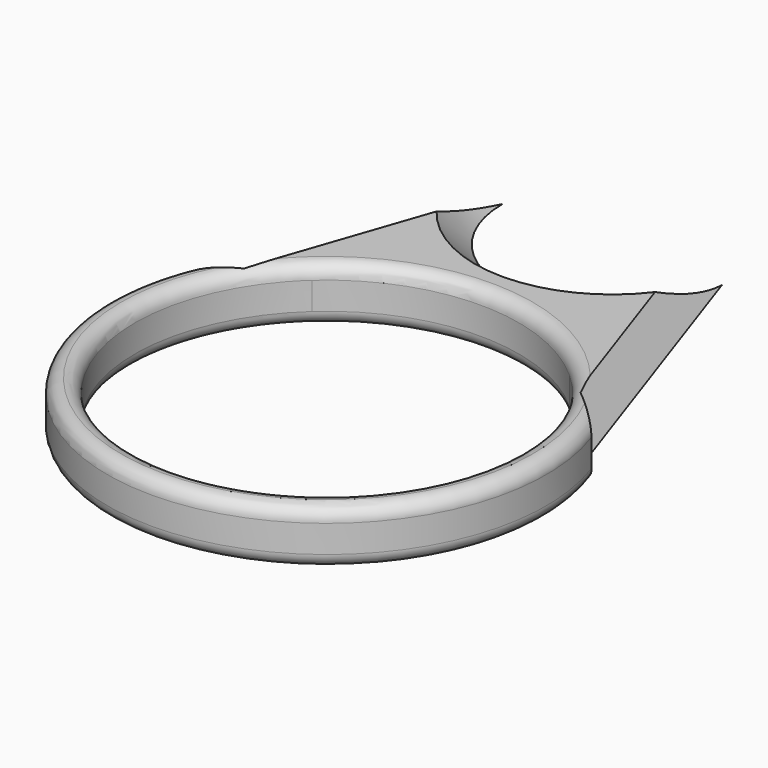
from build123d import *

# Parameters (mm, degrees)
F1_DEPTH    = 3.175
F2_SIZE     = 1.58749
F3_DEPTH    = 3.175
F4_T6_ANGLE = 235.7964191348
F4_T8_ANGLE = 235.7964191348


# Not quite as in the source:
# - a fillet or chamfer that OpenCascade refuses, or shapes differently, is made with other operations: its cross-section is extruded or revolved along the edge and cut away or added
# - a fillet or chamfer is up to 0.001 mm smaller than in the source, because OpenCascade refuses the exact size


with BuildPart() as f1:
    # F0 (on Top) → F1 (new body)
    with BuildSketch(Plane.XY):
        with BuildLine():
            ThreePointArc((-7.4530411175, 8.2425623656), (0, 11.1125), (7.4530411175, 8.2425623656))
            Line((7.4530411175, 8.2425623656), (12.0135135135, 4.1189189189))
            Line((12.0135135135, 4.1189189189), (6.35, 20.6375))
            ThreePointArc((6.35, 20.6375), (0, 14.2875), (-6.35, 20.6375))
            Line((-6.35, 20.6375), (-12.0135135135, 4.1189189189))
            Line((-12.0135135135, 4.1189189189), (-7.4530411175, 8.2425623656))
        make_face()
    extrude(amount=F1_DEPTH)

    # F2 (size 1.5875 in the source; OpenCascade refuses exactly that, so slightly less here)
    f2_edges = [f1.edges().sort_by_distance(p)[0] for p in [
        (-9.181757, 12.378209, 3.175),
        (-9.181757, 12.378209, 0),
        (0, 14.2875, 0),
        (0, 14.2875, 3.175),
        (9.181757, 12.378209, 3.175),
        (9.181757, 12.378209, 0),
    ]]
    chamfer(f2_edges, length=F2_SIZE)

    # F0 (on Top) → F3 (join)
    with BuildSketch(Plane.XY):
        with BuildLine():
            ThreePointArc((7.4530411175, 8.2425623656), (10.1565145515, 4.509198201), (11.1125, 0))
            ThreePointArc((11.1125, 0), (-4.509198201, -10.1565145515), (-7.4530411175, 8.2425623656))
            Line((-7.4530411175, 8.2425623656), (-12.0135135135, 4.1189189189))
            ThreePointArc((-12.0135135135, 4.1189189189), (0, -12.7), (12.0135135135, 4.1189189189))
            Line((12.0135135135, 4.1189189189), (7.4530411175, 8.2425623656))
        make_face()
    extrude(amount=F3_DEPTH)

    # F4: fillet of radius 0.79375 on 4 edges, made by hand

    # F4_s1 → F4_t2 (revolve, cut)
    with BuildSketch(Plane(origin=(0, 0, 0), x_dir=(0, 0, 1), z_dir=(-0.7417378957, -0.6706898643, 0))):
        with BuildLine():
            ThreePointArc((2.38125, 11.1125), (2.9425160076, 11.3449839924), (3.175, 11.90625))
            Line((3.175, 11.90625), (3.175, 11.1125))
            Line((3.175, 11.1125), (2.38125, 11.1125))
        make_face()
    revolve(axis=Axis((0, 0, 3.175), (0, 0, -1)), mode=Mode.SUBTRACT)

    # F4_s3 → F4_t4 (revolve, cut)
    with BuildSketch(Plane(origin=(0, 0, 0), x_dir=(0, 0, 1), z_dir=(0.7417378957, 0.6706898643, 0))):
        with BuildLine():
            ThreePointArc((0, -11.90625), (0.2324839924, -11.3449839924), (0.79375, -11.1125))
            Line((0.79375, -11.1125), (0, -11.1125))
            Line((0, -11.1125), (0, -11.90625))
        make_face()
    revolve(axis=Axis((0, 0, 0), (0, 0, 1)), mode=Mode.SUBTRACT)

    # F4_s5 → F4_t6 (revolve, cut)
    with BuildSketch(Plane(origin=(0, 0, 0), x_dir=(0, 0, 1), z_dir=(0.4679021973, 0.883780252, 0))):
        with BuildLine():
            ThreePointArc((0.79375, -12.7), (0.2324839924, -12.4675160076), (0, -11.90625))
            Line((0, -11.90625), (0, -12.7))
            Line((0, -12.7), (0.79375, -12.7))
        make_face()
    revolve(axis=Axis((0, 0, 0), (0, 0, 1)), revolution_arc=F4_T6_ANGLE, mode=Mode.SUBTRACT)

    # F4_s7 → F4_t8 (revolve, cut)
    with BuildSketch(Plane(origin=(0, 0, 0), x_dir=(0, 0, 1), z_dir=(0.4679021973, 0.883780252, 0))):
        with BuildLine():
            ThreePointArc((2.38125, -12.7), (2.9425160076, -12.4675160076), (3.175, -11.90625))
            Line((3.175, -11.90625), (3.175, -12.7))
            Line((3.175, -12.7), (2.38125, -12.7))
        make_face()
    revolve(axis=Axis((0, 0, 3.175), (0, 0, 1)), revolution_arc=F4_T8_ANGLE, mode=Mode.SUBTRACT)


solid = f1.part
